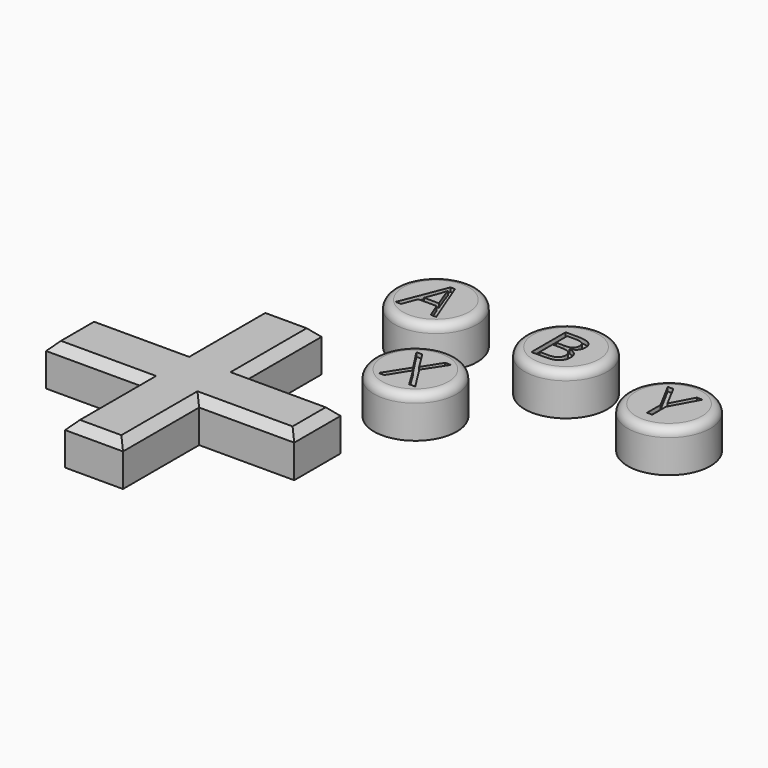
from build123d import *

# Parameters (mm, degrees)
F1_DEPTH      = 12.7
F2_SIZE       = 2.54
F3_R          = 12.7
F4_DEPTH      = 12.7
F5_TEXT_SIZE  = 19.6730821497
F6_DEPTH      = 1.27
F7_R          = 2.54
F8_TEXT_SIZE  = 18.4391004344
F9_DEPTH      = 1.27
F10_R         = 2.54
F11_TEXT_SIZE = 19.0523866978
F12_DEPTH     = 1.27
F13_TEXT_SIZE = 19.7531914132
F14_DEPTH     = 1.27
F15_R         = 2.54
F15_2_R       = 2.54


# Not quite as in the source:
# - Text() gives the source's letters only with a copy of the font that has no kerning and outlines rounded to 1/6400 em; it was checked with that copy


with BuildPart() as f1:
    # F0 (on Top) → F1 (new body)
    with BuildSketch(Plane.XY):
        Polygon((-37.2419713077, 8.89), (-37.2419713077, 0), (-37.2419713077, -8.89), (-8.0319713077, -8.89), (-8.0319713077, -38.1), (9.7480286923, -38.1), (9.7480286923, -8.89), (38.9580286923, -8.89), (38.9580286923, 0), (38.9580286923, 8.89), (9.7480286923, 8.89), (9.7480286923, 38.1), (-8.0319713077, 38.1), (-8.0319713077, 8.89), align=None)
    extrude(amount=F1_DEPTH)

    # F2
    f2_edges = [f1.edges().sort_by_distance(p)[0] for p in [
        (-37.241971, 0, 12.7),
        (-22.636971, -8.89, 12.7),
        (-8.031971, -23.495, 12.7),
        (0.858029, -38.1, 12.7),
        (9.748029, -23.495, 12.7),
        (24.353029, -8.89, 12.7),
        (38.958029, 0, 12.7),
        (24.353029, 8.89, 12.7),
        (9.748029, 23.495, 12.7),
        (0.858029, 38.1, 12.7),
        (-8.031971, 23.495, 12.7),
        (-22.636971, 8.89, 12.7),
    ]]
    chamfer(f2_edges, length=F2_SIZE)


with BuildPart() as f4:
    # F3 (on Top) → F4 (new body)
    with BuildSketch(Plane.XY):
        with Locations((22.1598185599, 66.4772838354)):
            Circle(F3_R)
    extrude(amount=F4_DEPTH)

    # F5 (on face) → F6 (cut)
    with BuildSketch(Plane.XY.offset(12.7)):
        with Locations((15.3359696269, 59.5715865493)):
            Text('A', F5_TEXT_SIZE, font='Open Sans', text_align=(TextAlign.LEFT, TextAlign.BOTTOM))
    extrude(amount=-F6_DEPTH, mode=Mode.SUBTRACT)

    # F7
    f7_edges = [f4.edges().sort_by_distance(p)[0] for p in [
        (9.459819, 66.477284, 12.7),
    ]]
    fillet(f7_edges, radius=F7_R)


with BuildPart() as f4b:
    # F3 (on Top) → F4, piece 2 (new body)
    with BuildSketch(Plane.XY):
        with Locations((61.8624761701, 66.808141768)):
            Circle(F3_R)
    extrude(amount=F4_DEPTH)

    # F8 (on face) → F9 (cut)
    with BuildSketch(Plane.XY.offset(12.7)):
        with Locations((55.2035197616, 59.5518946648)):
            Text('B', F8_TEXT_SIZE, font='Open Sans', text_align=(TextAlign.LEFT, TextAlign.BOTTOM))
    extrude(amount=-F9_DEPTH, mode=Mode.SUBTRACT)

    # F10
    f10_edges = [f4b.edges().sort_by_distance(p)[0] for p in [
        (49.162476, 66.808142, 12.7),
    ]]
    fillet(f10_edges, radius=F10_R)


with BuildPart() as f4c:
    # F3 (on Top) → F4, piece 3 (new body)
    with BuildSketch(Plane.XY):
        with Locations((99.5799973607, 59.198461473)):
            Circle(F3_R)
    extrude(amount=F4_DEPTH)

    # F11 (on face) → F12 (cut)
    with BuildSketch(Plane.XY.offset(12.7)):
        with Locations((93.82519871, 52.2771775723)):
            Text('Y', F11_TEXT_SIZE, font='Open Sans', text_align=(TextAlign.LEFT, TextAlign.BOTTOM))
    extrude(amount=-F12_DEPTH, mode=Mode.SUBTRACT)

    # F15#2
    f15_2_edges = [f4c.edges().sort_by_distance(p)[0] for p in [
        (86.879997, 59.198461, 12.7),
    ]]
    fillet(f15_2_edges, radius=F15_2_R)


with BuildPart() as f4d:
    # F3 (on Top) → F4, piece 4 (new body)
    with BuildSketch(Plane.XY):
        with Locations((40.919393301, 35.1626165211)):
            Circle(F3_R)
    extrude(amount=F4_DEPTH)

    # F13 (on face) → F14 (cut)
    with BuildSketch(Plane.XY.offset(12.7)):
        with Locations((35.1244658232, 28.1962379813)):
            Text('X', F13_TEXT_SIZE, font='Open Sans', text_align=(TextAlign.LEFT, TextAlign.BOTTOM))
    extrude(amount=-F14_DEPTH, mode=Mode.SUBTRACT)

    # F15
    f15_edges = [f4d.edges().sort_by_distance(p)[0] for p in [
        (28.219393, 35.162617, 12.7),
    ]]
    fillet(f15_edges, radius=F15_R)


solid = Compound([f1.part, f4.part, f4b.part, f4c.part, f4d.part])
